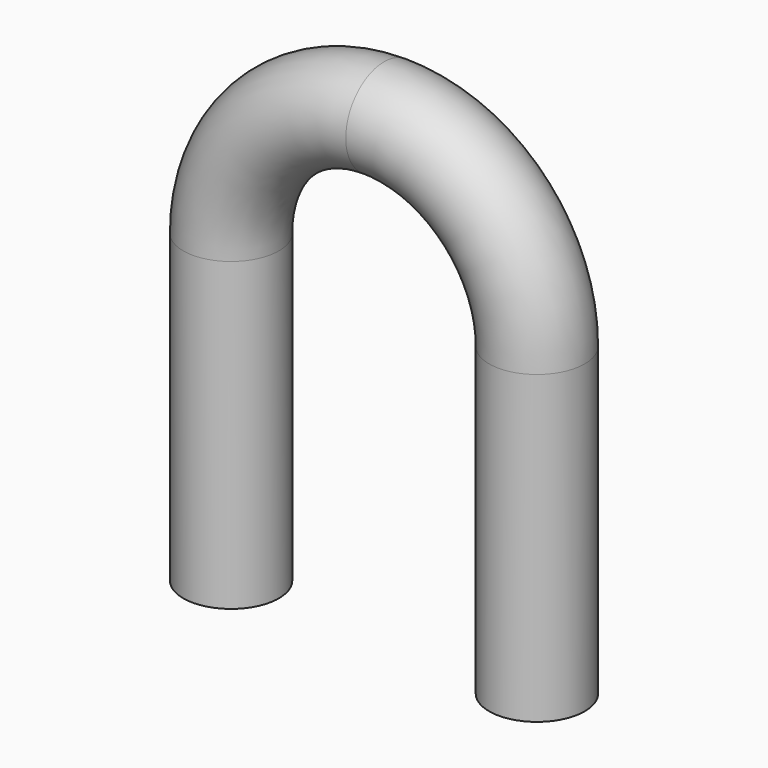
from build123d import *
from build123d import SkipClean  # not in build123d's __all__


with BuildPart() as f2:
    # F2: sweep along a path in F1
    with BuildLine(Plane.XZ) as f2_path:
        Line((25.4, 0), (25.4, 50.8))
        ThreePointArc((25.4, 50.8), (17.9605122421, 68.7605122421), (0, 76.2))
    # F0 (on Top) → F2 (sweep)
    with BuildSketch(Plane.XY):
        with BuildLine():
            ThreePointArc((17.4625, 0), (25.4, -7.9375), (33.3375, 0))
            ThreePointArc((33.3375, 0), (25.4, 7.9375), (17.4625, 0))
        make_face()
    sweep(path=f2_path.line)

    # F3: F2 across face


with BuildPart() as f2_1:
    add(f2.part, clean=False)
    with SkipClean():  # cleaning this boolean's faces spoils the solid; the shape is the same uncleaned
        add(f2.part.mirror(Plane(origin=(0, 0, 76.2), x_dir=(0, -1, 0), z_dir=(-1, 0, 0))), clean=False)


solid = f2_1.part
